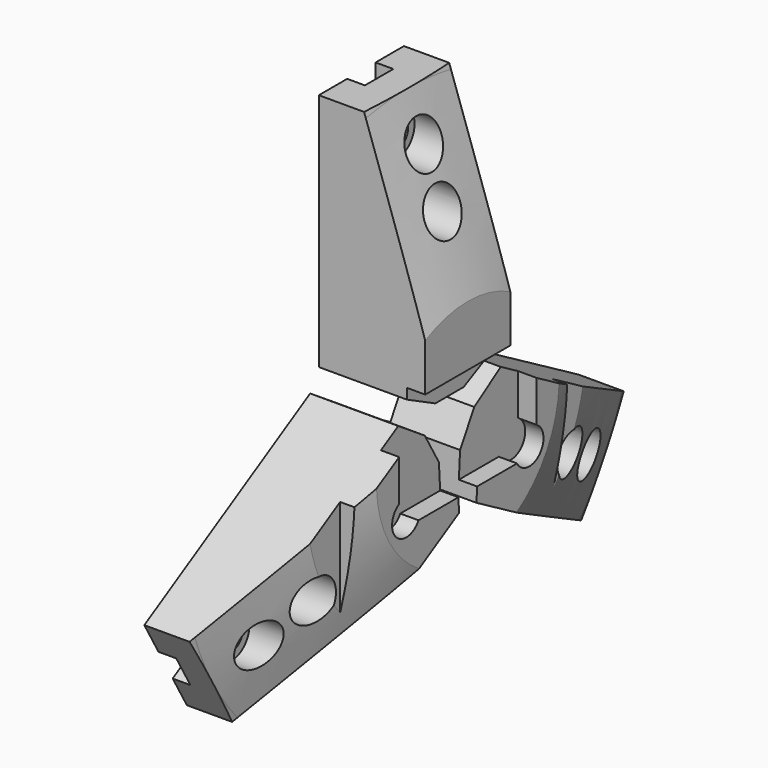
from build123d import *

# Parameters (mm, degrees)
F1_DEPTH  = 60
F2_R      = 8
F3_DEPTH  = 60
F2_R_2    = 12.5
F4_DEPTH  = 40
F6_DEPTH  = 145
F8_COUNT  = 3
F11_DEPTH = 10.3
F14_W     = 35
F14_H     = 60
F15_DEPTH = 105.6767622135


with BuildPart() as f1:
    # F0 (on Right) → F1 (new body)
    with BuildSketch(Plane.YZ):
        Polygon((-10, 14.39), (0, 14.39), (10, 14.39), (30, 24.39), (30, 159.39), (0, 159.39), (-30, 159.39), (-30, 24.39), align=None)
    extrude(amount=F1_DEPTH)

    # F2 (on face) → F3 (cut, through all)
    with BuildSketch(Plane.YZ.offset(60)):
        with Locations((0, 134.39)):
            Circle(F2_R)
        with Locations((0, 104.39)):
            Circle(F2_R)
    extrude(amount=-F3_DEPTH, mode=Mode.SUBTRACT)

    # F2 (on face) → F4 (cut)
    with BuildSketch(Plane.YZ.offset(60)):
        with Locations((0, 134.39)):
            Circle(F2_R_2)
        with Locations((0, 134.39)):
            Circle(F2_R, mode=Mode.SUBTRACT)
        with Locations((0, 104.39)):
            Circle(F2_R_2)
        with Locations((0, 104.39)):
            Circle(F2_R, mode=Mode.SUBTRACT)
    extrude(amount=-F4_DEPTH, mode=Mode.SUBTRACT)

    # F5 (on face) → F6 (cut, through all)
    with BuildSketch(Plane.XY.offset(159.39)):
        Polygon((0, 10), (0, 0), (0, -10), (10, -10), (10, 0), (10, 10), align=None)
    extrude(amount=-F6_DEPTH, mode=Mode.SUBTRACT)


with BuildPart() as f8_1:
    # F8: instance of F1
    add(f1.part.rotate(Axis((36.9910225272, 0, 0), (1, 0, 0)), 1 * 360 / F8_COUNT))


with BuildPart() as f8_2:
    # F8: instance of F1
    add(f1.part.rotate(Axis((36.9910225272, 0, 0), (1, 0, 0)), 2 * 360 / F8_COUNT))


with BuildPart() as f1_1:
    # F9: moved
    add(f1.part.moved(Location((3, 0, 0))))


with BuildPart() as f8_1_1:
    # F9: moved
    add(f8_1.part.moved(Location((3, 0, 0))))


with BuildPart() as f8_2_1:
    # F9: moved
    add(f8_2.part.moved(Location((3, 0, 0))))


with BuildPart() as f11_tool:
    # F10 (on face) → F11 (new body)
    with BuildSketch(Plane.YZ.offset(63)):
        with BuildLine():
            ThreePointArc((-48.375, -16.5897459622), (-50.4460678119, -32.3210678119), (-34.7147459622, -30.25))
            Line((-34.7147459622, -30.25), (34.7147459622, -30.25))
            ThreePointArc((34.7147459622, -30.25), (50.4460678119, -32.3210678119), (48.375, -16.5897459622))
            Line((48.375, -16.5897459622), (48.375, 16.5897459622))
            ThreePointArc((48.375, 16.5897459622), (50.4460678119, 32.3210678119), (34.7147459622, 30.25))
            Line((34.7147459622, 30.25), (30, 30.25))
            Line((30, 30.25), (30, 24.39))
            Line((30, 24.39), (10, 14.39))
            Line((10, 14.39), (-10, 14.39))
            Line((-10, 14.39), (-30, 24.39))
            Line((-30, 24.39), (-30, 30.25))
            Line((-30, 30.25), (-34.7147459622, 30.25))
            ThreePointArc((-34.7147459622, 30.25), (-50.4460678119, 32.3210678119), (-48.375, 16.5897459622))
            Line((-48.375, 16.5897459622), (-48.375, -16.5897459622))
        make_face()
        Polygon((30, 30.25), (-30, 30.25), (-30, 24.39), (-10, 14.39), (10, 14.39), (30, 24.39), align=None)
    extrude(amount=-F11_DEPTH)


with BuildPart() as f1_2:
    add(f1_1.part)

    # F11: cut by f11_tool
    add(f11_tool.part, mode=Mode.SUBTRACT)


with BuildPart() as f8_1_2:
    add(f8_1_1.part)

    # F11: cut by f11_tool
    add(f11_tool.part, mode=Mode.SUBTRACT)


with BuildPart() as f8_2_2:
    add(f8_2_1.part)

    # F11: cut by f11_tool
    add(f11_tool.part, mode=Mode.SUBTRACT)


with BuildPart() as f13_tool:
    # F12 (on Front) → F13 (revolve)
    with BuildSketch(Plane.XZ):
        Polygon((63, 159.39), (29.5, 159.39), (63, 64.39), align=None)
        Polygon((28.0894736842, 163.39), (29.5, 159.39), (63, 159.39), (63, 163.39), align=None)
    revolve(axis=Axis((30.98609671, 0, 0), (1, 0, 0)))


with BuildPart() as f1_3:
    add(f1_2.part)

    # F13: cut by f13_tool
    add(f13_tool.part, mode=Mode.SUBTRACT)


with BuildPart() as f8_1_3:
    add(f8_1_2.part)

    # F13: cut by f13_tool
    add(f13_tool.part, mode=Mode.SUBTRACT)


with BuildPart() as f8_2_3:
    add(f8_2_2.part)

    # F13: cut by f13_tool
    add(f13_tool.part, mode=Mode.SUBTRACT)


with BuildPart() as f15_tool:
    # F14 (on Top) → F15 (new body, through all)
    with BuildSketch(Plane.XY):
        with Locations((68.5, 105)):
            Rectangle(F14_W, F14_H)
        with Locations((68.5, -105)):
            Rectangle(F14_W, F14_H)
    extrude(amount=-F15_DEPTH)


with BuildPart() as f8_1_4:
    add(f8_1_3.part)

    # F15: cut by f15_tool
    add(f15_tool.part, mode=Mode.SUBTRACT)


with BuildPart() as f8_2_4:
    add(f8_2_3.part)

    # F15: cut by f15_tool
    add(f15_tool.part, mode=Mode.SUBTRACT)


solid = Compound([f1_3.part, f8_1_4.part, f8_2_4.part])
